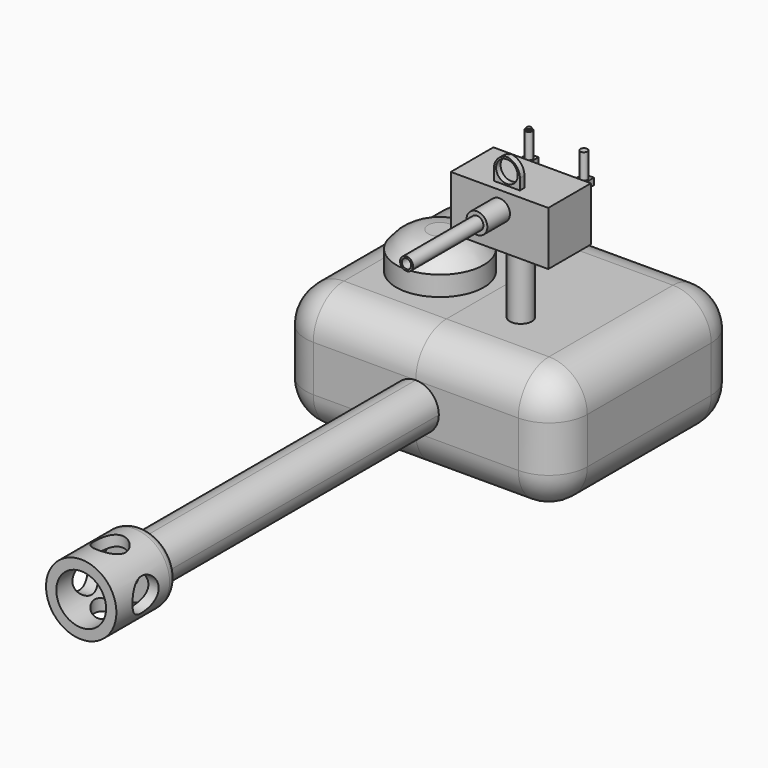
from build123d import *

# Parameters (mm, degrees)
F0_W          = 18.2884614915
F0_H          = 73.9338546991
F1_DEPTH      = 28.4915585071
F2_DEPTH      = 18.1708801538
F3_T1_DEPTH   = 100.3821844353
F5_W          = 27.3489970714
F5_H          = 77.689322154
F5_W_2        = 9.1442307457
F6_DEPTH      = 15.5535358936
F7_T1_DEPTH   = 120.9467486617
F8_W          = 36.4932278171
F8_H          = 38.844661077
F9_DEPTH      = 10.9388325363
F10_T1_DEPTH  = 344.5853614943
F11_T1_DEPTH  = 236.421989331
F12_R         = 5.08
F13_T1_DEPTH  = 77.689322154
F13_T4_ANGLE  = 126.7283433301
F13_T6_ANGLE  = 126.7283433301
F13_T8_ANGLE  = 126.7283433301
F13_T10_ANGLE = 126.7283433301
F14_T1_DEPTH  = 77.689322154
F14_T4_ANGLE  = 126.7283433301
F14_T6_ANGLE  = 126.7283433301
F14_T8_ANGLE  = 126.7283433301
F14_T10_ANGLE = 126.7283433301
F16_W         = 18.6711102724
F16_H         = 30.703663826
F17_DEPTH     = 16.2718910724
F18_R         = 5.08
F21_DEPTH     = 45.2075973153
F22_R         = 4.6669302811
F23_DEPTH     = 10.2340914309
F24_R         = 3.3014724235
F25_DEPTH     = 7.6366490684
F26_R         = 1.4543406252
F27_DEPTH     = 68.8959285617
F28_R         = 4.4727052122
F29_DEPTH     = 11.7008965462
F30_R         = 2.6235896832
F31_DEPTH     = 44.9183806777
F32_R         = 1.7763300942
F33_DEPTH     = 40.2182564139
F35_R         = 0.7381029721
F36_DEPTH     = 6.4580095932
F37_R         = 1.2103238767
F38_DEPTH     = 3.0198656023
F41_R         = 1.4634559334
F42_DEPTH     = 9.1732684523
F43_W         = 12.9226781428
F43_H         = 7.0590823889
F43_R         = 1.4634559334
F44_DEPTH     = 7.1371328086
F45_R         = 1.3829152172
F46_DEPTH     = 3.7461016327
F47_R         = 0.8584224563
F48_DEPTH     = 11.6643859074
F49_W         = 1.3765394688
F49_H         = 0.8871108294
F49_W_2       = 1.3459511101
F50_DEPTH     = 3.022047691
F51_R         = 0.4731491176
F51_R_2       = 0.4712154352
F52_DEPTH     = 3.2964972779
F53_R         = 0.2704180807
F54_DEPTH     = 0.2560240682
F55_R         = 0.6226984047
F56_DEPTH     = 16.576025635
F58_R         = 2.0357093932
F59_DEPTH     = 44.9477061629
F61_R         = 2.1758818467
F62_DEPTH     = 41.9628992677
F63_R         = 1.4299091098
F64_R         = 1.049613476
F65_W         = 3.4503787756
F65_H         = 0.7528178394
F66_DEPTH     = 3.3705015667
F67_T1_DEPTH  = 10.421244841
F68_R         = 1.4324717667
F69_DEPTH     = 40.5652821064
F70_R         = 5.8004176902
F71_DEPTH     = 2.6176106185
F72_R         = 5.8004176902
F73_DEPTH     = 2.2655753419


# Not quite as in the source:
# - a fillet or chamfer that OpenCascade refuses, or shapes differently, is made with other operations: its cross-section is extruded or revolved along the edge and cut away or added


with BuildPart() as f1:
    # F0 (on Top) → F1 (new body)
    with BuildSketch(Plane.XY):
        with Locations((36.4932278171, -0.1255981624)):
            Rectangle(F0_W, F0_H)
    extrude(amount=F1_DEPTH)

    # F2 (add): a face of the model
    f2_faces = [f1.faces().sort_by_distance(p)[0] for p in [
        (36.4932278171, -37.092525512, 14.2457792535),
    ]]
    extrude(f2_faces, amount=F2_DEPTH)

    # F3: fillet of radius 16.4187445888 on 2 edges, made by hand

    # F3_s2 → F3_t1 (cut)
    with BuildSketch(Plane.YZ.offset(-13.6978644005)):
        with BuildLine():
            ThreePointArc((-55.2634056658, 16.4187445888), (-50.4544667143, 4.8089389515), (-38.844661077, 0))
            Line((-38.844661077, 0), (-55.2634056658, 0))
            Line((-55.2634056658, 0), (-55.2634056658, 16.4187445888))
        make_face()
        with BuildLine():
            ThreePointArc((-38.844661077, 28.4915585071), (-50.4544667143, 23.6826195556), (-55.2634056658, 12.0728139183))
            Line((-55.2634056658, 12.0728139183), (-55.2634056658, 28.4915585071))
            Line((-55.2634056658, 28.4915585071), (-38.844661077, 28.4915585071))
        make_face()
    extrude(amount=F3_T1_DEPTH, mode=Mode.SUBTRACT)

    # F4: F1 across plane


with BuildPart() as f1_1:
    add(f1.part)
    add(f1.part.mirror(Plane.XZ))

    # F13: fillet of radius 5.08 on 2 edges, made by hand

    # F13_s2 → F13_t1 (cut)
    with BuildSketch(Plane.XZ.offset(-38.844661077)):
        with BuildLine():
            ThreePointArc((45.6374585629, 5.08), (44.1495610113, 1.4878975516), (40.5574585629, 0))
            Line((40.5574585629, 0), (45.6374585629, 0))
            Line((45.6374585629, 0), (45.6374585629, 5.08))
        make_face()
        with BuildLine():
            ThreePointArc((45.6374585629, 23.4115585071), (44.1495610113, 27.0036609555), (40.5574585629, 28.4915585071))
            Line((40.5574585629, 28.4915585071), (45.6374585629, 28.4915585071))
            Line((45.6374585629, 28.4915585071), (45.6374585629, 23.4115585071))
        make_face()
    extrude(amount=F13_T1_DEPTH, mode=Mode.SUBTRACT)

    # F13_s3 → F13_t4 (revolve, cut)
    with BuildSketch(Plane(origin=(0, 19.6785427541, 26.3735524772), x_dir=(1, 0, 0), z_dir=(0, -0.5980216998, -0.8014799103))):
        with BuildLine():
            ThreePointArc((45.6374585629, -35.2521553639), (44.1495610113, -38.8442578124), (40.5574585629, -40.3321553639))
            Line((40.5574585629, -40.3321553639), (45.6374585629, -40.3321553639))
            Line((45.6374585629, -40.3321553639), (45.6374585629, -35.2521553639))
        make_face()
    revolve(axis=Axis((45.6374585629, 38.844661077, 12.0728139183), (1, 0, 0)), revolution_arc=F13_T4_ANGLE, mode=Mode.SUBTRACT)

    # F13_s5 → F13_t6 (revolve, cut)
    with BuildSketch(Plane.XZ.offset(-38.844661077)):
        with BuildLine():
            ThreePointArc((45.6374585629, 5.08), (44.1495610113, 1.4878975516), (40.5574585629, 0))
            Line((40.5574585629, 0), (45.6374585629, 0))
            Line((45.6374585629, 0), (45.6374585629, 5.08))
        make_face()
    revolve(axis=Axis((45.6374585629, 38.844661077, 16.4187445888), (1, 0, 0)), revolution_arc=F13_T6_ANGLE, mode=Mode.SUBTRACT)

    # F13_s7 → F13_t8 (revolve, cut)
    with BuildSketch(Plane.XZ.offset(38.844661077)):
        with BuildLine():
            ThreePointArc((45.6374585629, 5.08), (44.1495610113, 1.4878975516), (40.5574585629, 0))
            Line((40.5574585629, 0), (45.6374585629, 0))
            Line((45.6374585629, 0), (45.6374585629, 5.08))
        make_face()
    revolve(axis=Axis((45.6374585629, -38.844661077, 16.4187445888), (-1, 0, 0)), revolution_arc=F13_T8_ANGLE, mode=Mode.SUBTRACT)

    # F13_s9 → F13_t10 (revolve, cut)
    with BuildSketch(Plane(origin=(0, -19.6785427541, 26.3735524772), x_dir=(1, 0, 0), z_dir=(0, 0.5980216998, -0.8014799103))):
        with BuildLine():
            ThreePointArc((45.6374585629, 35.2521553639), (44.1495610113, 38.8442578124), (40.5574585629, 40.3321553639))
            Line((40.5574585629, 40.3321553639), (45.6374585629, 40.3321553639))
            Line((45.6374585629, 40.3321553639), (45.6374585629, 35.2521553639))
        make_face()
    revolve(axis=Axis((45.6374585629, -38.844661077, 12.0728139183), (-1, 0, 0)), revolution_arc=F13_T10_ANGLE, mode=Mode.SUBTRACT)

    # F14: fillet of radius 5.08 on 2 edges, made by hand

    # F14_s2 → F14_t1 (cut)
    with BuildSketch(Plane.XZ.offset(-38.844661077)):
        with BuildLine():
            ThreePointArc((32.4289970714, 0), (28.836894623, 1.4878975516), (27.3489970714, 5.08))
            Line((27.3489970714, 5.08), (27.3489970714, 0))
            Line((27.3489970714, 0), (32.4289970714, 0))
        make_face()
        with BuildLine():
            ThreePointArc((32.4289970714, 28.4915585071), (28.836894623, 27.0036609555), (27.3489970714, 23.4115585071))
            Line((27.3489970714, 23.4115585071), (27.3489970714, 28.4915585071))
            Line((27.3489970714, 28.4915585071), (32.4289970714, 28.4915585071))
        make_face()
    extrude(amount=F14_T1_DEPTH, mode=Mode.SUBTRACT)

    # F14_s3 → F14_t4 (revolve, cut)
    with BuildSketch(Plane(origin=(0, 19.6785427541, 26.3735524772), x_dir=(1, 0, 0), z_dir=(0, -0.5980216998, -0.8014799103))):
        with BuildLine():
            ThreePointArc((32.4289970714, -40.3321553639), (28.836894623, -38.8442578124), (27.3489970714, -35.2521553639))
            Line((27.3489970714, -35.2521553639), (27.3489970714, -40.3321553639))
            Line((27.3489970714, -40.3321553639), (32.4289970714, -40.3321553639))
        make_face()
    revolve(axis=Axis((27.3489970714, 38.844661077, 12.0728139183), (1, 0, 0)), revolution_arc=F14_T4_ANGLE, mode=Mode.SUBTRACT)

    # F14_s5 → F14_t6 (revolve, cut)
    with BuildSketch(Plane.XZ.offset(-38.844661077)):
        with BuildLine():
            ThreePointArc((32.4289970714, 0), (28.836894623, 1.4878975516), (27.3489970714, 5.08))
            Line((27.3489970714, 5.08), (27.3489970714, 0))
            Line((27.3489970714, 0), (32.4289970714, 0))
        make_face()
    revolve(axis=Axis((27.3489970714, 38.844661077, 16.4187445888), (1, 0, 0)), revolution_arc=F14_T6_ANGLE, mode=Mode.SUBTRACT)

    # F14_s7 → F14_t8 (revolve, cut)
    with BuildSketch(Plane.XZ.offset(38.844661077)):
        with BuildLine():
            ThreePointArc((32.4289970714, 0), (28.836894623, 1.4878975516), (27.3489970714, 5.08))
            Line((27.3489970714, 5.08), (27.3489970714, 0))
            Line((27.3489970714, 0), (32.4289970714, 0))
        make_face()
    revolve(axis=Axis((27.3489970714, -38.844661077, 16.4187445888), (-1, 0, 0)), revolution_arc=F14_T8_ANGLE, mode=Mode.SUBTRACT)

    # F14_s9 → F14_t10 (revolve, cut)
    with BuildSketch(Plane(origin=(0, -19.6785427541, 26.3735524772), x_dir=(1, 0, 0), z_dir=(0, 0.5980216998, -0.8014799103))):
        with BuildLine():
            ThreePointArc((32.4289970714, 40.3321553639), (28.836894623, 38.8442578124), (27.3489970714, 35.2521553639))
            Line((27.3489970714, 35.2521553639), (27.3489970714, 40.3321553639))
            Line((27.3489970714, 40.3321553639), (32.4289970714, 40.3321553639))
        make_face()
    revolve(axis=Axis((27.3489970714, -38.844661077, 12.0728139183), (-1, 0, 0)), revolution_arc=F14_T10_ANGLE, mode=Mode.SUBTRACT)


with BuildPart() as f6:
    # F5 (on face) → F6 (new body)
    with BuildSketch(Plane.XY.offset(28.4915585071)):
        with Locations((13.6744985357, 0)):
            Rectangle(F5_W, F5_H)
        with Locations((31.9211124443, 0)):
            Rectangle(F5_W_2, F5_H)
    extrude(amount=F6_DEPTH)

    # F7: fillet of radius 16.8907041689 on 1 edges, made by hand

    # F7_s2 → F7_t1 (cut)
    with BuildSketch(Plane.YZ.offset(-42.2267604223)):
        with BuildLine():
            ThreePointArc((-38.844661077, 27.1543902317), (-33.8974883649, 39.0979216886), (-21.9539569081, 44.0450944006))
            Line((-21.9539569081, 44.0450944006), (-38.844661077, 44.0450944006))
            Line((-38.844661077, 44.0450944006), (-38.844661077, 27.1543902317))
        make_face()
    extrude(amount=F7_T1_DEPTH, mode=Mode.SUBTRACT)

    # F8 (on face) → F9 (join)
    with BuildSketch(Plane.XY.offset(44.0450944006)):
        with Locations((18.2466139086, 19.4223305385)):
            Rectangle(F8_W, F8_H)
    extrude(amount=F9_DEPTH)

    # F10: fillet of radius 179.017667452 on 1 edges, made by hand

    # F10_s2 → F10_t1 (cut)
    with BuildSketch(Plane.YZ.offset(-154.0460668386)):
        with BuildLine():
            ThreePointArc((0, 44.0450944006), (30.3274992539, 52.2280055256), (61.6184267354, 54.983926937))
            Line((61.6184267354, 54.983926937), (0, 54.983926937))
            Line((0, 54.983926937), (0, 44.0450944006))
        make_face()
    extrude(amount=F10_T1_DEPTH, mode=Mode.SUBTRACT)

    # F11: fillet of radius 28.9687689723 on 1 edges, made by hand

    # F11_s2 → F11_t1 (cut)
    with BuildSketch(Plane.YZ.offset(-99.9643807569)):
        with BuildLine():
            ThreePointArc((0, 44.0450944006), (26.5056416367, 40.5317813704), (38.844661077, 16.8117264322))
            Line((38.844661077, 16.8117264322), (39.4240364564, 16.8117264322))
            Line((39.4240364564, 16.8117264322), (39.4240364564, 53.5294337574))
            Line((39.4240364564, 53.5294337574), (38.770955731, 54.1041017939))
            ThreePointArc((38.770955731, 54.1041017939), (19.0192706965, 50.4380615005), (-0.1975178421, 44.58976176))
            Line((-0.1975178421, 44.58976176), (0, 44.0450944006))
        make_face()
    extrude(amount=F11_T1_DEPTH, mode=Mode.SUBTRACT)

    # F12
    f12_edges = [f6.edges().sort_by_distance(p)[0] for p in [
        (36.493228, -33.414982, 39.561678),
        (36.493228, 21.262292, 43.448909),
    ]]
    fillet(f12_edges, radius=F12_R)


with BuildPart() as f17:
    # F16 (on offset) → F17 (new body)
    with BuildSketch(Plane.XY.offset(47.5083142519)):
        with Locations((9.3355551362, 5.1864385605)):
            Rectangle(F16_W, F16_H)
    extrude(amount=F17_DEPTH)

    # F18
    f18_edges = [f17.edges().sort_by_distance(p)[0] for p in [
        (18.67111, 5.186439, 63.780205),
        (18.67111, 20.53827, 55.64426),
        (18.67111, 5.186439, 47.508314),
        (18.67111, -10.165393, 55.64426),
        (9.335555, 20.53827, 63.780205),
        (9.335555, 20.53827, 47.508314),
        (9.335555, -10.165393, 63.780205),
        (9.335555, -10.165393, 47.508314),
    ]]
    fillet(f18_edges, radius=F18_R)


with BuildPart() as f19_1:
    # F19: instance of F17
    add(f17.part.mirror(Plane.YZ))

    # F35 (on face) → F36 (join)
    with BuildSketch(Plane.XY.offset(63.7802053243)):
        with Locations((-7.3755094782, 11.6158071905)):
            Circle(F35_R)
    extrude(amount=F36_DEPTH)

    # F37 (on face) → F38 (join)
    with BuildSketch(Plane.XY.offset(70.2382149175)):
        with Locations((-7.3755094782, 11.6158071905)):
            Circle(F37_R)
    extrude(amount=F38_DEPTH)

    # F64
    f64_edges = [f19_1.edges().sort_by_distance(p)[0] for p in [
        (-8.585833, 11.615807, 73.258081),
    ]]
    fillet(f64_edges, radius=F64_R)

    # F70 (on face) → F71 (join)
    with BuildSketch(Plane.XY.offset(63.7802053243)):
        with Locations((-7.1992054582, 2.8470307589)):
            Circle(F70_R)
    extrude(amount=F71_DEPTH)


with BuildPart() as f19_2:
    # F19: instance of F6
    add(f6.part.mirror(Plane.YZ))


with BuildPart() as f19_3:
    # F19: instance of F1
    add(f1_1.part.mirror(Plane.YZ))


with BuildPart() as f21:
    # F20 (on face) → F21 (new body)
    with BuildSketch(Plane.XZ.offset(10.1653933525)):
        with BuildLine():
            Line((0, 52.5883142519), (0, 58.7002053243))
            ThreePointArc((0, 58.7002053243), (-3.0559455362, 55.6442597881), (0, 52.5883142519))
        make_face()
        with BuildLine():
            ThreePointArc((0, 52.5883142519), (2.1608798116, 53.4833799765), (3.0559455362, 55.6442597881))
            ThreePointArc((3.0559455362, 55.6442597881), (2.1608798116, 57.8051395997), (0, 58.7002053243))
            Line((0, 58.7002053243), (0, 52.5883142519))
        make_face()
    extrude(amount=F21_DEPTH)

    # F22 (on face) → F23 (join)
    with BuildSketch(Plane.XZ.offset(55.3729906678)):
        with Locations((0, 55.6442597881)):
            Circle(F22_R)
    extrude(amount=F23_DEPTH)

    # F24 (on face) → F25 (cut)
    with BuildSketch(Plane.XZ.offset(65.6070820987)):
        with Locations((0, 55.6442597881)):
            Circle(F24_R)
    extrude(amount=-F25_DEPTH, mode=Mode.SUBTRACT)

    # F26 (on face) → F27 (cut)
    with BuildSketch(Plane.XZ.offset(57.9704330303)):
        with Locations((0, 55.6442597881)):
            Circle(F26_R)
    extrude(amount=-F27_DEPTH, mode=Mode.SUBTRACT)

    # F58 (on offset) → F59 (cut)
    with BuildSketch(Plane.XY.offset(60.7252959162)):
        with Locations((0, -60.8349591494)):
            Circle(F58_R)
    extrude(amount=-F59_DEPTH, mode=Mode.SUBTRACT)

    # F61 (on offset) → F62 (cut)
    with BuildSketch(Plane.YZ.offset(5.5607780814)):
        with Locations((-60.7723332942, 55.6115694344)):
            Circle(F61_R)
    extrude(amount=-F62_DEPTH, mode=Mode.SUBTRACT)

    # F63
    f63_edges = [f21.edges().sort_by_distance(p)[0] for p in [
        (-4.66693, -55.372991, 55.64426),
    ]]
    fillet(f63_edges, radius=F63_R)


with BuildPart() as f29:
    # F28 (on offset) → F29 (new body)
    with BuildSketch(Plane.XY.offset(47.5083142519)):
        Circle(F28_R)
    extrude(amount=-F29_DEPTH)


with BuildPart() as f6_1:
    add(f6.part)

    # F30 (on Front) → F31 (join)
    with BuildSketch(Plane.XZ):
        with Locations((18.8204254955, 31.8526290357)):
            Circle(F30_R)
    extrude(amount=-F31_DEPTH)

    # F32 (on face) → F33 (cut)
    with BuildSketch(Plane(origin=(0, 44.9183806777, 0), x_dir=(-1, 0, 0), z_dir=(0, 1, 0))):
        with Locations((-18.8204254955, 31.8526290357)):
            Circle(F32_R)
    extrude(amount=-F33_DEPTH, mode=Mode.SUBTRACT)


with BuildPart() as f17_1:
    add(f17.part)

    # F41 (on face) → F42 (join)
    with BuildSketch(Plane.XY.offset(63.7802053243)):
        with Locations((5.7961493731, 0)):
            Circle(F41_R)
    extrude(amount=F42_DEPTH)

    # F43 (on face) → F44 (join)
    with BuildSketch(Plane.XY.offset(72.9534737766)):
        with Locations((5.7961493731, 0)):
            Rectangle(F43_W, F43_H)
        with Locations((5.7961493731, 0)):
            Circle(F43_R, mode=Mode.SUBTRACT)
        with Locations((5.7961493731, 0)):
            Circle(F43_R)
    extrude(amount=F44_DEPTH)

    # F45 (on face) → F46 (join)
    with BuildSketch(Plane.XZ.offset(3.5295411944)):
        with Locations((5.7961493731, 77.7374729514)):
            Circle(F45_R)
    extrude(amount=F46_DEPTH)

    # F47 (on face) → F48 (join)
    with BuildSketch(Plane.XZ.offset(7.2756428272)):
        with Locations((5.7961493731, 77.7374729514)):
            Circle(F47_R)
    extrude(amount=F48_DEPTH)

    # F49 (on face) → F50 (join)
    with BuildSketch(Plane(origin=(0, 3.5295411944, 0), x_dir=(-1, 0, 0), z_dir=(0, 1, 0))):
        with Locations((-9.5428386703, 78.4232392907)):
            Rectangle(F49_W, F49_H)
        with Locations((-2.2318810225, 78.4232392907)):
            Rectangle(F49_W_2, F49_H)
    extrude(amount=F50_DEPTH)

    # F51 (on face) → F52 (join)
    with BuildSketch(Plane.XY.offset(78.8667947054)):
        with Locations((2.2582218517, 5.7621202432)):
            Circle(F51_R)
        with Locations((9.5428386703, 5.7621202432)):
            Circle(F51_R_2)
    extrude(amount=F52_DEPTH)

    # F55 (on face) → F56 (cut)
    with BuildSketch(Plane.XZ.offset(18.9400287345)):
        with Locations((5.7961493731, 77.7374729514)):
            Circle(F55_R)
    extrude(amount=-F56_DEPTH, mode=Mode.SUBTRACT)

    # F65 (on face) → F66 (join)
    with BuildSketch(Plane.XY.offset(80.0906065851)):
        with Locations((5.7961493731, -1.9382666796)):
            Rectangle(F65_W, F65_H)
    extrude(amount=F66_DEPTH)

    # F67: fillet of radius 1.9336854003 on 2 edges, made by hand

    # F67_s2 → F67_t1 (cut)
    with BuildSketch(Plane.XZ.offset(-3.2723557408)):
        with BuildLine():
            ThreePointArc((7.5213387609, 81.5274227515), (6.9549754198, 82.8947448108), (5.5876533605, 83.4611081518))
            Line((5.5876533605, 83.4611081518), (7.5213387609, 83.4611081518))
            Line((7.5213387609, 83.4611081518), (7.5213387609, 81.5274227515))
        make_face()
        with BuildLine():
            ThreePointArc((4.0709599853, 81.5274227515), (4.6373233263, 82.8947448108), (6.0046453856, 83.4611081518))
            Line((6.0046453856, 83.4611081518), (4.0709599853, 83.4611081518))
            Line((4.0709599853, 83.4611081518), (4.0709599853, 81.5274227515))
        make_face()
    extrude(amount=F67_T1_DEPTH, mode=Mode.SUBTRACT)

    # F68 (on face) → F69 (cut)
    with BuildSketch(Plane.XZ.offset(2.3146755993)):
        with Locations((5.7961493731, 81.7328095436)):
            Circle(F68_R)
    extrude(amount=-F69_DEPTH, mode=Mode.SUBTRACT)


with BuildPart() as f54:
    # F53 (on face) → F54 (new body)
    with BuildSketch(Plane.XY.offset(82.1632919833)):
        with Locations((2.2582218517, 5.7621202432)):
            Circle(F53_R)
    extrude(amount=F54_DEPTH)


with BuildPart() as f73:
    # F72 (on face) → F73 (new body)
    with BuildSketch(Plane.XY.offset(66.3978159428)):
        with Locations((-7.1992054582, 2.8470307589)):
            Circle(F72_R)
    extrude(amount=F73_DEPTH)

    # F74: fillet of radius 5.08 on 1 edges, made by hand

    # F74_s1 → F74_t2 (revolve, cut)
    with BuildSketch(Plane.XZ.offset(-2.8470307589)):
        with BuildLine():
            ThreePointArc((-1.398787768, 66.3978159428), (-3.2290361028, 68.0613192242), (-5.627902787, 68.6633912846))
            Line((-5.627902787, 68.6633912846), (-1.398787768, 68.6633912846))
            Line((-1.398787768, 68.6633912846), (-1.398787768, 66.3978159428))
        make_face()
    revolve(axis=Axis((-7.1992054582, 2.8470307589, 68.6633912846), (0, 0, 1)), mode=Mode.SUBTRACT)


solid = Compound([f19_1.part, f21.part, f17_1.part, f54.part, f73.part])
